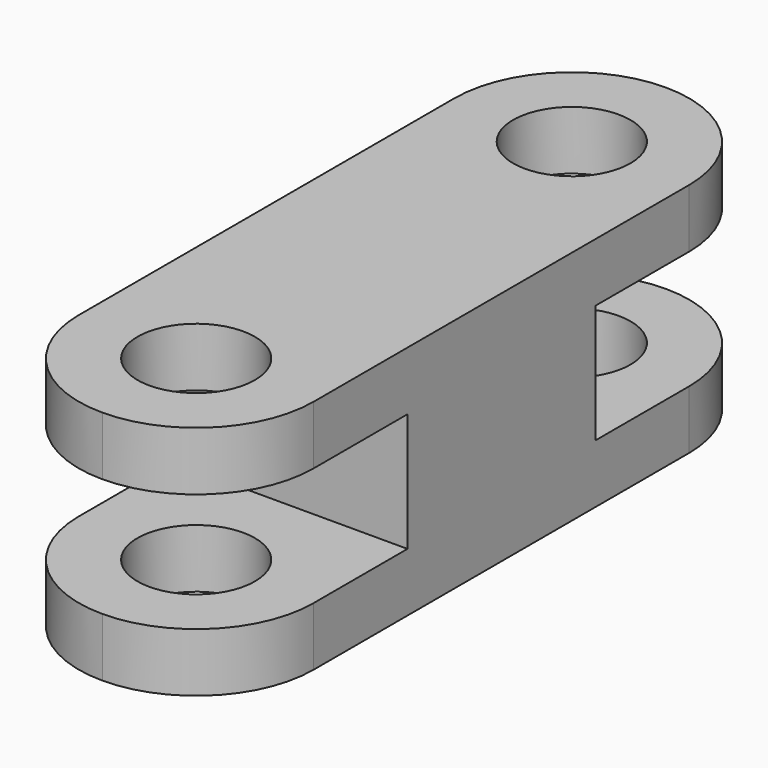
from build123d import *

# Parameters (mm, degrees)
F0_W     = 40
F0_H     = 80
F1_DEPTH = 20.1
F2_R     = 10
F3_DEPTH = 10
F5_W     = 40
F5_H     = 20.2
F6_DEPTH = 20
F7_R     = 10
F8_DEPTH = 25
F9_R     = 19.99999


# Not quite as in the source:
# - a fillet or chamfer is up to 0.001 mm smaller than in the source, because OpenCascade refuses the exact size


with BuildPart() as f1:
    # F0 (on Top) → F1 (new body)
    with BuildSketch(Plane.XY):
        Rectangle(F0_W, F0_H)
    extrude(amount=F1_DEPTH)

    # F2 (on face) → F3 (join)
    with BuildSketch(Plane.XY.offset(20.1)):
        with BuildLine():
            Line((-20, 60), (-20, 40))
            Line((-20, 40), (20, 40))
            Line((20, 40), (20, 60))
            ThreePointArc((20, 60), (0, 80), (-20, 60))
        make_face()
        with Locations((0, 60)):
            Circle(F2_R, mode=Mode.SUBTRACT)
    extrude(amount=-F3_DEPTH)

    # F4: F1 across plane


with BuildPart() as f1_1:
    add(f1.part)
    add(f1.part.mirror(Plane.XY))

    # F5 (on Right) → F6 (cut, symmetric)
    with BuildSketch(Plane.YZ):
        with Locations((-20, 0)):
            Rectangle(F5_W, F5_H)
    extrude(amount=F6_DEPTH, both=True, mode=Mode.SUBTRACT)

    # F7 (on Top) → F8 (cut, symmetric)
    with BuildSketch(Plane.XY):
        with Locations((0, -20)):
            Circle(F7_R)
    extrude(amount=F8_DEPTH, both=True, mode=Mode.SUBTRACT)

    # F9 (radius 20 in the source; OpenCascade refuses exactly that, so slightly less here)
    f9_edges = [f1_1.edges().sort_by_distance(p)[0] for p in [
        (20, -40, -15.1),
        (-20, -40, -15.1),
        (-20, -40, 15.1),
        (20, -40, 15.1),
    ]]
    fillet(f9_edges, radius=F9_R)


solid = f1_1.part
